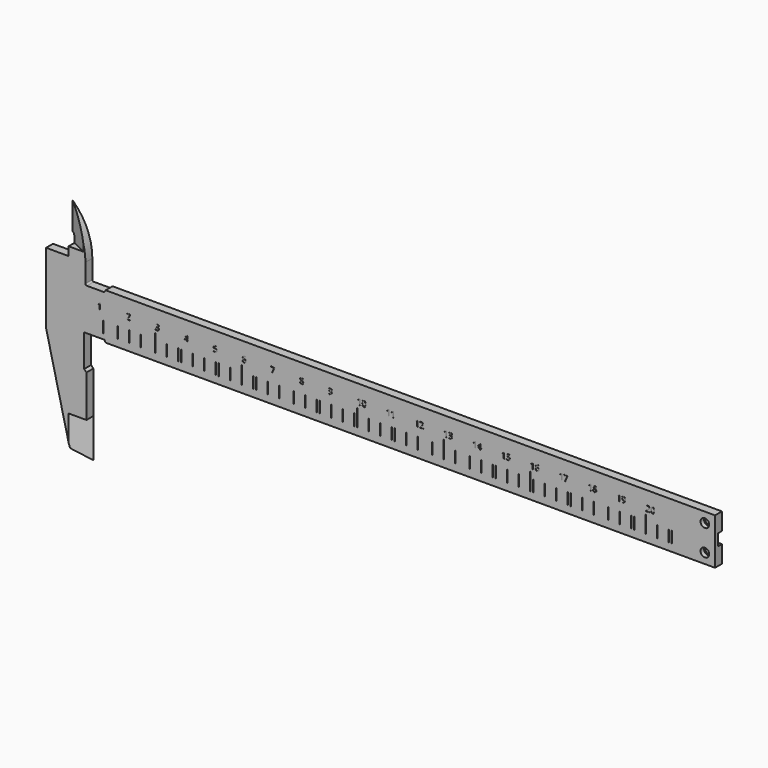
from build123d import *

# Parameters (mm, degrees)
F1_DEPTH      = 3
F2_R          = 1.5
F3_DEPTH      = 1.5
F4_R          = 1
F5_DEPTH      = 3.001
F8_DEPTH      = 12.5
F9_W          = 1.65
F9_H          = 4
F10_DEPTH     = 210
F13_DEPTH     = 13.5
F14_W         = 0.05
F14_H         = 6
F14_H_2       = 4
F15_DEPTH     = 0.1
F16_TEXT_SIZE = 2.7777777778
F17_DEPTH     = 0.1


# Not quite as in the source:
# - Text() gives the source's letters only with a copy of the font that has no kerning and outlines rounded to 1/6400 em; it was checked with that copy


with BuildPart() as f1:
    # F0 (on Front) → F1 (new body)
    with BuildSketch(Plane.XZ):
        with BuildLine():
            Line((0, 0), (0, 8))
            Line((0, 8), (-211.2, 8))
            Line((-211.2, 8), (-211.6330127019, 7.25))
            Line((-211.6330127019, 7.25), (-217.7016400172, 7.25))
            ThreePointArc((-217.7016400172, 7.25), (-218.0551934078, 7.3964466094), (-218.2016400172, 7.75))
            Line((-218.2016400172, 7.75), (-218.2016400172, 14.25))
            ThreePointArc((-218.2016400172, 14.25), (-219.9852255022, 22.7193218849), (-225.0330127019, 29.75))
            Line((-225.0330127019, 29.75), (-225.0330127019, 20.25))
            ThreePointArc((-225.0330127019, 20.25), (-224.3259059207, 19.9571067812), (-224.0330127019, 19.25))
            Line((-224.0330127019, 19.25), (-224.0330127019, 14.25))
            Line((-224.0330127019, 14.25), (-231.8330127019, 14.25))
            Line((-231.8330127019, 14.25), (-231.8330127019, -10.25))
            Line((-231.8330127019, -10.25), (-223.6330127019, -44.2947523929))
            Line((-223.6330127019, -44.2947523929), (-217.8330127019, -47.25))
            Line((-217.8330127019, -47.25), (-217.8330127019, -19.25))
            Line((-217.8330127019, -19.25), (-218.6330127019, -18.45))
            Line((-218.6330127019, -18.45), (-218.6330127019, -7.25))
            Line((-218.6330127019, -7.25), (-211.6330127019, -7.25))
            Line((-211.6330127019, -7.25), (-211.2, -8))
            Line((-211.2, -8), (0, -8))
            Line((0, -8), (0, 0))
        make_face()
    extrude(amount=F1_DEPTH)

    # F2 (on face) → F3 (cut)
    with BuildSketch(Plane.XZ.offset(3)):
        with Locations((-3.5, 4.5)):
            Circle(F2_R)
        with Locations((-3.5, -4.5)):
            Circle(F2_R)
    extrude(amount=-F3_DEPTH, mode=Mode.SUBTRACT)

    # F4 (on Front) → F5 (cut, through all)
    with BuildSketch(Plane.XZ):
        with Locations((-3.5, 4.5)):
            Circle(F4_R)
        with Locations((-3.5, -4.5)):
            Circle(F4_R)
    extrude(amount=F5_DEPTH, mode=Mode.SUBTRACT)

    # F7 (on plane+point) → F8 (cut)
    with BuildSketch(Plane.XY.offset(29.75)):
        Polygon((-225.0330127019, 0), (-225.0330127019, -3), (-218.8821011772, -3), align=None)
    extrude(amount=-F8_DEPTH, mode=Mode.SUBTRACT)

    # F9 (on face) → F10 (cut)
    with BuildSketch(Plane.YZ):
        with Locations((-0.825, 0)):
            Rectangle(F9_W, F9_H)
    extrude(amount=-F10_DEPTH, mode=Mode.SUBTRACT)

    # F12 (on plane+point) → F13 (cut)
    with BuildSketch(Plane(origin=(0, 0, -47.25), x_dir=(1, 0, 0), z_dir=(0, 0, -1))):
        Polygon((-217.8330127019, 0), (-217.8330127019, 3), (-223.9839242266, 3), align=None)
    extrude(amount=-F13_DEPTH, mode=Mode.SUBTRACT)

    # F14 (on face) → F15 (cut)
    with BuildSketch(Plane.XZ.offset(3)):
        with Locations((-214.0080127019, -2.5)):
            Rectangle(F14_W, F14_H)
        with Locations((-204.0080127019, -2.5)):
            Rectangle(F14_W, F14_H)
        with Locations((-194.0080127019, -2.5)):
            Rectangle(F14_W, F14_H)
        with Locations((-184.0080127019, -2.5)):
            Rectangle(F14_W, F14_H)
        with Locations((-174.0080127019, -2.5)):
            Rectangle(F14_W, F14_H)
        with Locations((-164.0080127019, -2.5)):
            Rectangle(F14_W, F14_H)
        with Locations((-154.0080127019, -2.5)):
            Rectangle(F14_W, F14_H)
        with Locations((-144.0080127019, -2.5)):
            Rectangle(F14_W, F14_H)
        with Locations((-134.0080127019, -2.5)):
            Rectangle(F14_W, F14_H)
        with Locations((-124.0080127019, -2.5)):
            Rectangle(F14_W, F14_H)
        with Locations((-114.0080127019, -2.5)):
            Rectangle(F14_W, F14_H)
        with Locations((-104.0080127019, -2.5)):
            Rectangle(F14_W, F14_H)
        with Locations((-94.0080127019, -2.5)):
            Rectangle(F14_W, F14_H)
        with Locations((-84.0080127019, -2.5)):
            Rectangle(F14_W, F14_H)
        with Locations((-74.0080127019, -2.5)):
            Rectangle(F14_W, F14_H)
        with Locations((-64.0080127019, -2.5)):
            Rectangle(F14_W, F14_H)
        with Locations((-54.0080127019, -2.5)):
            Rectangle(F14_W, F14_H)
        with Locations((-44.0080127019, -2.5)):
            Rectangle(F14_W, F14_H)
        with Locations((-34.0080127019, -2.5)):
            Rectangle(F14_W, F14_H)
        with Locations((-24.0080127019, -2.5)):
            Rectangle(F14_W, F14_H)
        with Locations((-213.0080127019, -3.5)):
            Rectangle(F14_W, F14_H_2)
        with Locations((-212.0080127019, -3.5)):
            Rectangle(F14_W, F14_H_2)
        with Locations((-211.0080127019, -3.5)):
            Rectangle(F14_W, F14_H_2)
        with Locations((-210.0080127019, -3.5)):
            Rectangle(F14_W, F14_H_2)
        with Locations((-209.0080127019, -3.5)):
            Rectangle(F14_W, F14_H_2)
        with Locations((-208.0080127019, -3.5)):
            Rectangle(F14_W, F14_H_2)
        with Locations((-207.0080127019, -3.5)):
            Rectangle(F14_W, F14_H_2)
        with Locations((-206.0080127019, -3.5)):
            Rectangle(F14_W, F14_H_2)
        with Locations((-205.0080127019, -3.5)):
            Rectangle(F14_W, F14_H_2)
        with Locations((-202.0080127019, -3.5)):
            Rectangle(F14_W, F14_H_2)
        with Locations((-198.0080127019, -3.5)):
            Rectangle(F14_W, F14_H_2)
        with Locations((-203.0080127019, -3.5)):
            Rectangle(F14_W, F14_H_2)
        with Locations((-197.0080127019, -3.5)):
            Rectangle(F14_W, F14_H_2)
        with Locations((-201.0080127019, -3.5)):
            Rectangle(F14_W, F14_H_2)
        with Locations((-200.0080127019, -3.5)):
            Rectangle(F14_W, F14_H_2)
        with Locations((-196.0080127019, -3.5)):
            Rectangle(F14_W, F14_H_2)
        with Locations((-195.0080127019, -3.5)):
            Rectangle(F14_W, F14_H_2)
        with Locations((-199.0080127019, -3.5)):
            Rectangle(F14_W, F14_H_2)
        with Locations((-192.0080127019, -3.5)):
            Rectangle(F14_W, F14_H_2)
        with Locations((-188.0080127019, -3.5)):
            Rectangle(F14_W, F14_H_2)
        with Locations((-193.0080127019, -3.5)):
            Rectangle(F14_W, F14_H_2)
        with Locations((-187.0080127019, -3.5)):
            Rectangle(F14_W, F14_H_2)
        with Locations((-191.0080127019, -3.5)):
            Rectangle(F14_W, F14_H_2)
        with Locations((-190.0080127019, -3.5)):
            Rectangle(F14_W, F14_H_2)
        with Locations((-186.0080127019, -3.5)):
            Rectangle(F14_W, F14_H_2)
        with Locations((-185.0080127019, -3.5)):
            Rectangle(F14_W, F14_H_2)
        with Locations((-189.0080127019, -3.5)):
            Rectangle(F14_W, F14_H_2)
        with Locations((-182.0080127019, -3.5)):
            Rectangle(F14_W, F14_H_2)
        with Locations((-178.0080127019, -3.5)):
            Rectangle(F14_W, F14_H_2)
        with Locations((-183.0080127019, -3.5)):
            Rectangle(F14_W, F14_H_2)
        with Locations((-177.0080127019, -3.5)):
            Rectangle(F14_W, F14_H_2)
        with Locations((-181.0080127019, -3.5)):
            Rectangle(F14_W, F14_H_2)
        with Locations((-180.0080127019, -3.5)):
            Rectangle(F14_W, F14_H_2)
        with Locations((-176.0080127019, -3.5)):
            Rectangle(F14_W, F14_H_2)
        with Locations((-175.0080127019, -3.5)):
            Rectangle(F14_W, F14_H_2)
        with Locations((-179.0080127019, -3.5)):
            Rectangle(F14_W, F14_H_2)
        with Locations((-172.0080127019, -3.5)):
            Rectangle(F14_W, F14_H_2)
        with Locations((-168.0080127019, -3.5)):
            Rectangle(F14_W, F14_H_2)
        with Locations((-173.0080127019, -3.5)):
            Rectangle(F14_W, F14_H_2)
        with Locations((-167.0080127019, -3.5)):
            Rectangle(F14_W, F14_H_2)
        with Locations((-171.0080127019, -3.5)):
            Rectangle(F14_W, F14_H_2)
        with Locations((-170.0080127019, -3.5)):
            Rectangle(F14_W, F14_H_2)
        with Locations((-166.0080127019, -3.5)):
            Rectangle(F14_W, F14_H_2)
        with Locations((-165.0080127019, -3.5)):
            Rectangle(F14_W, F14_H_2)
        with Locations((-169.0080127019, -3.5)):
            Rectangle(F14_W, F14_H_2)
        with Locations((-162.0080127019, -3.5)):
            Rectangle(F14_W, F14_H_2)
        with Locations((-158.0080127019, -3.5)):
            Rectangle(F14_W, F14_H_2)
        with Locations((-163.0080127019, -3.5)):
            Rectangle(F14_W, F14_H_2)
        with Locations((-157.0080127019, -3.5)):
            Rectangle(F14_W, F14_H_2)
        with Locations((-161.0080127019, -3.5)):
            Rectangle(F14_W, F14_H_2)
        with Locations((-160.0080127019, -3.5)):
            Rectangle(F14_W, F14_H_2)
        with Locations((-156.0080127019, -3.5)):
            Rectangle(F14_W, F14_H_2)
        with Locations((-155.0080127019, -3.5)):
            Rectangle(F14_W, F14_H_2)
        with Locations((-159.0080127019, -3.5)):
            Rectangle(F14_W, F14_H_2)
        with Locations((-152.0080127019, -3.5)):
            Rectangle(F14_W, F14_H_2)
        with Locations((-148.0080127019, -3.5)):
            Rectangle(F14_W, F14_H_2)
        with Locations((-153.0080127019, -3.5)):
            Rectangle(F14_W, F14_H_2)
        with Locations((-147.0080127019, -3.5)):
            Rectangle(F14_W, F14_H_2)
        with Locations((-151.0080127019, -3.5)):
            Rectangle(F14_W, F14_H_2)
        with Locations((-150.0080127019, -3.5)):
            Rectangle(F14_W, F14_H_2)
        with Locations((-146.0080127019, -3.5)):
            Rectangle(F14_W, F14_H_2)
        with Locations((-145.0080127019, -3.5)):
            Rectangle(F14_W, F14_H_2)
        with Locations((-149.0080127019, -3.5)):
            Rectangle(F14_W, F14_H_2)
        with Locations((-142.0080127019, -3.5)):
            Rectangle(F14_W, F14_H_2)
        with Locations((-138.0080127019, -3.5)):
            Rectangle(F14_W, F14_H_2)
        with Locations((-143.0080127019, -3.5)):
            Rectangle(F14_W, F14_H_2)
        with Locations((-137.0080127019, -3.5)):
            Rectangle(F14_W, F14_H_2)
        with Locations((-141.0080127019, -3.5)):
            Rectangle(F14_W, F14_H_2)
        with Locations((-140.0080127019, -3.5)):
            Rectangle(F14_W, F14_H_2)
        with Locations((-136.0080127019, -3.5)):
            Rectangle(F14_W, F14_H_2)
        with Locations((-135.0080127019, -3.5)):
            Rectangle(F14_W, F14_H_2)
        with Locations((-139.0080127019, -3.5)):
            Rectangle(F14_W, F14_H_2)
        with Locations((-132.0080127019, -3.5)):
            Rectangle(F14_W, F14_H_2)
        with Locations((-128.0080127019, -3.5)):
            Rectangle(F14_W, F14_H_2)
        with Locations((-133.0080127019, -3.5)):
            Rectangle(F14_W, F14_H_2)
        with Locations((-127.0080127019, -3.5)):
            Rectangle(F14_W, F14_H_2)
        with Locations((-131.0080127019, -3.5)):
            Rectangle(F14_W, F14_H_2)
        with Locations((-130.0080127019, -3.5)):
            Rectangle(F14_W, F14_H_2)
        with Locations((-126.0080127019, -3.5)):
            Rectangle(F14_W, F14_H_2)
        with Locations((-125.0080127019, -3.5)):
            Rectangle(F14_W, F14_H_2)
        with Locations((-129.0080127019, -3.5)):
            Rectangle(F14_W, F14_H_2)
        with Locations((-122.0080127019, -3.5)):
            Rectangle(F14_W, F14_H_2)
        with Locations((-118.0080127019, -3.5)):
            Rectangle(F14_W, F14_H_2)
        with Locations((-123.0080127019, -3.5)):
            Rectangle(F14_W, F14_H_2)
        with Locations((-117.0080127019, -3.5)):
            Rectangle(F14_W, F14_H_2)
        with Locations((-121.0080127019, -3.5)):
            Rectangle(F14_W, F14_H_2)
        with Locations((-120.0080127019, -3.5)):
            Rectangle(F14_W, F14_H_2)
        with Locations((-116.0080127019, -3.5)):
            Rectangle(F14_W, F14_H_2)
        with Locations((-115.0080127019, -3.5)):
            Rectangle(F14_W, F14_H_2)
        with Locations((-119.0080127019, -3.5)):
            Rectangle(F14_W, F14_H_2)
        with Locations((-112.0080127019, -3.5)):
            Rectangle(F14_W, F14_H_2)
        with Locations((-108.0080127019, -3.5)):
            Rectangle(F14_W, F14_H_2)
        with Locations((-113.0080127019, -3.5)):
            Rectangle(F14_W, F14_H_2)
        with Locations((-107.0080127019, -3.5)):
            Rectangle(F14_W, F14_H_2)
        with Locations((-111.0080127019, -3.5)):
            Rectangle(F14_W, F14_H_2)
        with Locations((-110.0080127019, -3.5)):
            Rectangle(F14_W, F14_H_2)
        with Locations((-106.0080127019, -3.5)):
            Rectangle(F14_W, F14_H_2)
        with Locations((-105.0080127019, -3.5)):
            Rectangle(F14_W, F14_H_2)
        with Locations((-109.0080127019, -3.5)):
            Rectangle(F14_W, F14_H_2)
        with Locations((-102.0080127019, -3.5)):
            Rectangle(F14_W, F14_H_2)
        with Locations((-98.0080127019, -3.5)):
            Rectangle(F14_W, F14_H_2)
        with Locations((-103.0080127019, -3.5)):
            Rectangle(F14_W, F14_H_2)
        with Locations((-97.0080127019, -3.5)):
            Rectangle(F14_W, F14_H_2)
        with Locations((-101.0080127019, -3.5)):
            Rectangle(F14_W, F14_H_2)
        with Locations((-100.0080127019, -3.5)):
            Rectangle(F14_W, F14_H_2)
        with Locations((-96.0080127019, -3.5)):
            Rectangle(F14_W, F14_H_2)
        with Locations((-95.0080127019, -3.5)):
            Rectangle(F14_W, F14_H_2)
        with Locations((-99.0080127019, -3.5)):
            Rectangle(F14_W, F14_H_2)
        with Locations((-92.0080127019, -3.5)):
            Rectangle(F14_W, F14_H_2)
        with Locations((-88.0080127019, -3.5)):
            Rectangle(F14_W, F14_H_2)
        with Locations((-93.0080127019, -3.5)):
            Rectangle(F14_W, F14_H_2)
        with Locations((-87.0080127019, -3.5)):
            Rectangle(F14_W, F14_H_2)
        with Locations((-91.0080127019, -3.5)):
            Rectangle(F14_W, F14_H_2)
        with Locations((-90.0080127019, -3.5)):
            Rectangle(F14_W, F14_H_2)
        with Locations((-86.0080127019, -3.5)):
            Rectangle(F14_W, F14_H_2)
        with Locations((-85.0080127019, -3.5)):
            Rectangle(F14_W, F14_H_2)
        with Locations((-89.0080127019, -3.5)):
            Rectangle(F14_W, F14_H_2)
        with Locations((-82.0080127019, -3.5)):
            Rectangle(F14_W, F14_H_2)
        with Locations((-78.0080127019, -3.5)):
            Rectangle(F14_W, F14_H_2)
        with Locations((-83.0080127019, -3.5)):
            Rectangle(F14_W, F14_H_2)
        with Locations((-77.0080127019, -3.5)):
            Rectangle(F14_W, F14_H_2)
        with Locations((-81.0080127019, -3.5)):
            Rectangle(F14_W, F14_H_2)
        with Locations((-80.0080127019, -3.5)):
            Rectangle(F14_W, F14_H_2)
        with Locations((-76.0080127019, -3.5)):
            Rectangle(F14_W, F14_H_2)
        with Locations((-75.0080127019, -3.5)):
            Rectangle(F14_W, F14_H_2)
        with Locations((-79.0080127019, -3.5)):
            Rectangle(F14_W, F14_H_2)
        with Locations((-72.0080127019, -3.5)):
            Rectangle(F14_W, F14_H_2)
        with Locations((-68.0080127019, -3.5)):
            Rectangle(F14_W, F14_H_2)
        with Locations((-73.0080127019, -3.5)):
            Rectangle(F14_W, F14_H_2)
        with Locations((-67.0080127019, -3.5)):
            Rectangle(F14_W, F14_H_2)
        with Locations((-71.0080127019, -3.5)):
            Rectangle(F14_W, F14_H_2)
        with Locations((-70.0080127019, -3.5)):
            Rectangle(F14_W, F14_H_2)
        with Locations((-66.0080127019, -3.5)):
            Rectangle(F14_W, F14_H_2)
        with Locations((-65.0080127019, -3.5)):
            Rectangle(F14_W, F14_H_2)
        with Locations((-69.0080127019, -3.5)):
            Rectangle(F14_W, F14_H_2)
        with Locations((-62.0080127019, -3.5)):
            Rectangle(F14_W, F14_H_2)
        with Locations((-58.0080127019, -3.5)):
            Rectangle(F14_W, F14_H_2)
        with Locations((-63.0080127019, -3.5)):
            Rectangle(F14_W, F14_H_2)
        with Locations((-57.0080127019, -3.5)):
            Rectangle(F14_W, F14_H_2)
        with Locations((-61.0080127019, -3.5)):
            Rectangle(F14_W, F14_H_2)
        with Locations((-60.0080127019, -3.5)):
            Rectangle(F14_W, F14_H_2)
        with Locations((-56.0080127019, -3.5)):
            Rectangle(F14_W, F14_H_2)
        with Locations((-55.0080127019, -3.5)):
            Rectangle(F14_W, F14_H_2)
        with Locations((-59.0080127019, -3.5)):
            Rectangle(F14_W, F14_H_2)
        with Locations((-52.0080127019, -3.5)):
            Rectangle(F14_W, F14_H_2)
        with Locations((-48.0080127019, -3.5)):
            Rectangle(F14_W, F14_H_2)
        with Locations((-53.0080127019, -3.5)):
            Rectangle(F14_W, F14_H_2)
        with Locations((-47.0080127019, -3.5)):
            Rectangle(F14_W, F14_H_2)
        with Locations((-51.0080127019, -3.5)):
            Rectangle(F14_W, F14_H_2)
        with Locations((-50.0080127019, -3.5)):
            Rectangle(F14_W, F14_H_2)
        with Locations((-46.0080127019, -3.5)):
            Rectangle(F14_W, F14_H_2)
        with Locations((-45.0080127019, -3.5)):
            Rectangle(F14_W, F14_H_2)
        with Locations((-49.0080127019, -3.5)):
            Rectangle(F14_W, F14_H_2)
        with Locations((-42.0080127019, -3.5)):
            Rectangle(F14_W, F14_H_2)
        with Locations((-38.0080127019, -3.5)):
            Rectangle(F14_W, F14_H_2)
        with Locations((-43.0080127019, -3.5)):
            Rectangle(F14_W, F14_H_2)
        with Locations((-37.0080127019, -3.5)):
            Rectangle(F14_W, F14_H_2)
        with Locations((-41.0080127019, -3.5)):
            Rectangle(F14_W, F14_H_2)
        with Locations((-40.0080127019, -3.5)):
            Rectangle(F14_W, F14_H_2)
        with Locations((-36.0080127019, -3.5)):
            Rectangle(F14_W, F14_H_2)
        with Locations((-35.0080127019, -3.5)):
            Rectangle(F14_W, F14_H_2)
        with Locations((-39.0080127019, -3.5)):
            Rectangle(F14_W, F14_H_2)
        with Locations((-32.0080127019, -3.5)):
            Rectangle(F14_W, F14_H_2)
        with Locations((-28.0080127019, -3.5)):
            Rectangle(F14_W, F14_H_2)
        with Locations((-33.0080127019, -3.5)):
            Rectangle(F14_W, F14_H_2)
        with Locations((-27.0080127019, -3.5)):
            Rectangle(F14_W, F14_H_2)
        with Locations((-31.0080127019, -3.5)):
            Rectangle(F14_W, F14_H_2)
        with Locations((-30.0080127019, -3.5)):
            Rectangle(F14_W, F14_H_2)
        with Locations((-26.0080127019, -3.5)):
            Rectangle(F14_W, F14_H_2)
        with Locations((-25.0080127019, -3.5)):
            Rectangle(F14_W, F14_H_2)
        with Locations((-29.0080127019, -3.5)):
            Rectangle(F14_W, F14_H_2)
        with Locations((-22.0080127019, -3.5)):
            Rectangle(F14_W, F14_H_2)
        with Locations((-18.0080127019, -3.5)):
            Rectangle(F14_W, F14_H_2)
        with Locations((-23.0080127019, -3.5)):
            Rectangle(F14_W, F14_H_2)
        with Locations((-17.0080127019, -3.5)):
            Rectangle(F14_W, F14_H_2)
        with Locations((-21.0080127019, -3.5)):
            Rectangle(F14_W, F14_H_2)
        with Locations((-20.0080127019, -3.5)):
            Rectangle(F14_W, F14_H_2)
        with Locations((-16.0080127019, -3.5)):
            Rectangle(F14_W, F14_H_2)
        with Locations((-15.0080127019, -3.5)):
            Rectangle(F14_W, F14_H_2)
        with Locations((-19.0080127019, -3.5)):
            Rectangle(F14_W, F14_H_2)
    extrude(amount=-F15_DEPTH, mode=Mode.SUBTRACT)

    # F16 (on face) → F17 (cut)
    with BuildSketch(Plane.XZ.offset(3)):
        with Locations((-213.9830127019, 1.5)):
            Text('1', F16_TEXT_SIZE, font='Open Sans', text_align=(TextAlign.LEFT, TextAlign.BOTTOM))
        with Locations((-203.9830127019, 1.5)):
            Text('2', F16_TEXT_SIZE, font='Open Sans', text_align=(TextAlign.LEFT, TextAlign.BOTTOM))
        with Locations((-193.9830127019, 1.5)):
            Text('3', F16_TEXT_SIZE, font='Open Sans', text_align=(TextAlign.LEFT, TextAlign.BOTTOM))
        with Locations((-183.9830127019, 1.5)):
            Text('4', F16_TEXT_SIZE, font='Open Sans', text_align=(TextAlign.LEFT, TextAlign.BOTTOM))
        with Locations((-173.9830127019, 1.5)):
            Text('5', F16_TEXT_SIZE, font='Open Sans', text_align=(TextAlign.LEFT, TextAlign.BOTTOM))
        with Locations((-163.9830127019, 1.5)):
            Text('6', F16_TEXT_SIZE, font='Open Sans', text_align=(TextAlign.LEFT, TextAlign.BOTTOM))
        with Locations((-153.9830127019, 1.5)):
            Text('7', F16_TEXT_SIZE, font='Open Sans', text_align=(TextAlign.LEFT, TextAlign.BOTTOM))
        with Locations((-143.9830127019, 1.5)):
            Text('8', F16_TEXT_SIZE, font='Open Sans', text_align=(TextAlign.LEFT, TextAlign.BOTTOM))
        with Locations((-133.9830127019, 1.5)):
            Text('9', F16_TEXT_SIZE, font='Open Sans', text_align=(TextAlign.LEFT, TextAlign.BOTTOM))
        with Locations((-123.9830127019, 1.5)):
            Text('10', F16_TEXT_SIZE, font='Open Sans', text_align=(TextAlign.LEFT, TextAlign.BOTTOM))
        with Locations((-113.9830127019, 1.5)):
            Text('11', F16_TEXT_SIZE, font='Open Sans', text_align=(TextAlign.LEFT, TextAlign.BOTTOM))
        with Locations((-103.9830127019, 1.5)):
            Text('12', F16_TEXT_SIZE, font='Open Sans', text_align=(TextAlign.LEFT, TextAlign.BOTTOM))
        with Locations((-93.9830127019, 1.5)):
            Text('13', F16_TEXT_SIZE, font='Open Sans', text_align=(TextAlign.LEFT, TextAlign.BOTTOM))
        with Locations((-83.9830127019, 1.5)):
            Text('14', F16_TEXT_SIZE, font='Open Sans', text_align=(TextAlign.LEFT, TextAlign.BOTTOM))
        with Locations((-73.9830127019, 1.5)):
            Text('15', F16_TEXT_SIZE, font='Open Sans', text_align=(TextAlign.LEFT, TextAlign.BOTTOM))
        with Locations((-63.9830127019, 1.5)):
            Text('16', F16_TEXT_SIZE, font='Open Sans', text_align=(TextAlign.LEFT, TextAlign.BOTTOM))
        with Locations((-53.9830127019, 1.5)):
            Text('17', F16_TEXT_SIZE, font='Open Sans', text_align=(TextAlign.LEFT, TextAlign.BOTTOM))
        with Locations((-43.9830127019, 1.5)):
            Text('18', F16_TEXT_SIZE, font='Open Sans', text_align=(TextAlign.LEFT, TextAlign.BOTTOM))
        with Locations((-33.9830127019, 1.5)):
            Text('19', F16_TEXT_SIZE, font='Open Sans', text_align=(TextAlign.LEFT, TextAlign.BOTTOM))
        with Locations((-23.9830127019, 1.5)):
            Text('20', F16_TEXT_SIZE, font='Open Sans', text_align=(TextAlign.LEFT, TextAlign.BOTTOM))
    extrude(amount=-F17_DEPTH, mode=Mode.SUBTRACT)


solid = f1.part
